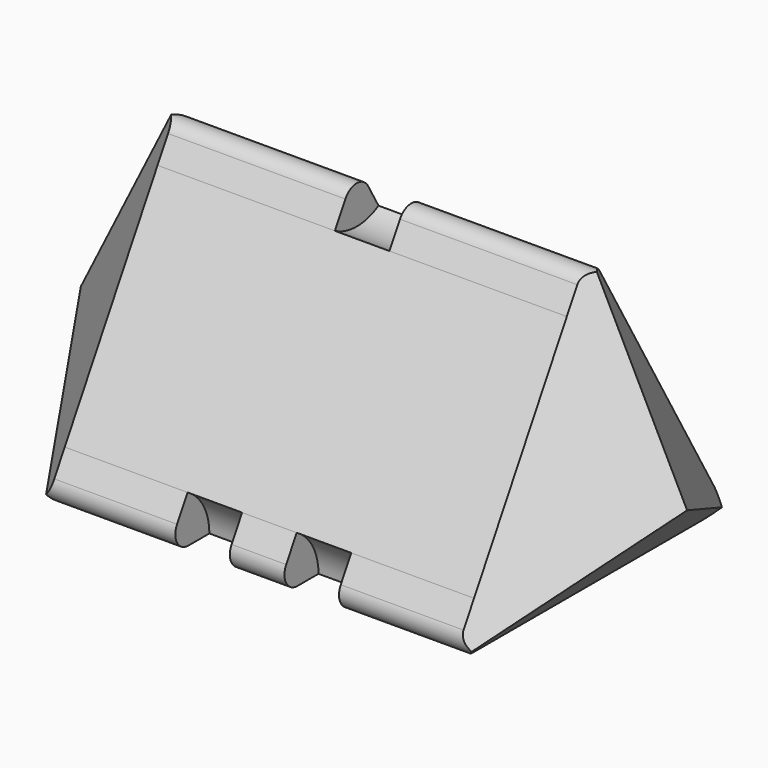
from build123d import *

# Parameters (mm, degrees)
F1_DEPTH    = 15
F4_T1_DEPTH = 20.1961524227
F5_START    = 6.5
F5_DEPTH    = 2
F6_START    = 4.5
F6_DEPTH    = 2
F7_START    = 8.5
F7_DEPTH    = 2
F8_START    = 2.5
F8_DEPTH    = 2
F9_START    = 6.5
F9_DEPTH    = 2
F10_START   = 10.5
F10_DEPTH   = 2


# Not quite as in the source:
# - a fillet or chamfer that OpenCascade refuses, or shapes differently, is made with other operations: its cross-section is extruded or revolved along the edge and cut away or added
# - an extrude whose draft closes it to a point is written as a loft to that point
# - a feature names something its author has since deleted; it is built from what else it names


with BuildPart() as f1:
    # F0 (on Right) → F1 (new body)
    with BuildSketch(Plane.YZ):
        with BuildLine():
            Line((4.25, 2.1650635095), (6.25, 2.1650635095))
            Line((6.25, 2.1650635095), (5.25, 3.897114317))
            ThreePointArc((5.25, 3.897114317), (4.5179491924, 3.1650635095), (4.25, 2.1650635095))
        make_face()
        with BuildLine():
            ThreePointArc((4.25, 2.1650635095), (4.5179491924, 3.1650635095), (5.25, 3.897114317))
            Line((5.25, 3.897114317), (1, 11.2583302492))
            ThreePointArc((1, 11.2583302492), (0, 10.9903810568), (-1, 11.2583302492))
            Line((-1, 11.2583302492), (-5.25, 3.897114317))
            ThreePointArc((-5.25, 3.897114317), (-4.5179491924, 3.1650635095), (-4.25, 2.1650635095))
            Line((-4.25, 2.1650635095), (4.25, 2.1650635095))
        make_face()
        with BuildLine():
            ThreePointArc((-1, 11.2583302492), (0, 10.9903810568), (1, 11.2583302492))
            Line((1, 11.2583302492), (0, 12.9903810568))
            Line((0, 12.9903810568), (-1, 11.2583302492))
        make_face()
        with BuildLine():
            Line((-6.25, 2.1650635095), (-4.25, 2.1650635095))
            ThreePointArc((-4.25, 2.1650635095), (-4.5179491924, 3.1650635095), (-5.25, 3.897114317))
            Line((-5.25, 3.897114317), (-6.25, 2.1650635095))
        make_face()
    extrude(amount=F1_DEPTH)

    # F1_face (on face) → F2 section 0
    with BuildSketch(Plane(origin=(0, 0, 5.7735026919), x_dir=(0, 1, 0), z_dir=(-1, 0, 0)), mode=Mode.PRIVATE) as f2_s0:
        Polygon((0, -7.2168783649), (6.25, 3.6084391824), (-6.25, 3.6084391824), align=None)
    loft([f2_s0.sketch, Vertex(-3.6084391824, 0, 5.7735026919)], ruled=True)

    # F1_face1 (on face) → F3 section 0
    with BuildSketch(Plane(origin=(15, 0, 5.7735026919), x_dir=(0, 1, 0), z_dir=(1, 0, 0)), mode=Mode.PRIVATE) as f3_s0:
        Polygon((6.25, -3.6084391824), (0, 7.2168783649), (-6.25, -3.6084391824), align=None)
    loft([f3_s0.sketch, Vertex(18.6084391824, 0, 5.7735026919)], ruled=True)

    # F4: fillet of radius 0.6 on 3 edges, made by hand

    # F4_s2 → F4_t1 (cut)
    with BuildSketch(Plane.YZ.offset(-2.5980762114)):
        with BuildLine():
            ThreePointArc((0.5196152423, 12.0903810568), (0, 12.3903810568), (-0.5196152423, 12.0903810568))
            Line((-0.5196152423, 12.0903810568), (0, 12.9903810568))
            Line((0, 12.9903810568), (0.5196152423, 12.0903810568))
        make_face()
        with BuildLine():
            ThreePointArc((-5.2107695155, 2.1650635095), (-5.7303847577, 2.4650635095), (-5.7303847577, 3.0650635095))
            Line((-5.7303847577, 3.0650635095), (-6.25, 2.1650635095))
            Line((-6.25, 2.1650635095), (-5.2107695155, 2.1650635095))
        make_face()
        with BuildLine():
            ThreePointArc((5.7303847577, 3.0650635095), (5.7303847577, 2.4650635095), (5.2107695155, 2.1650635095))
            Line((5.2107695155, 2.1650635095), (6.25, 2.1650635095))
            Line((6.25, 2.1650635095), (5.7303847577, 3.0650635095))
        make_face()
    extrude(amount=F4_T1_DEPTH, mode=Mode.SUBTRACT)

    # F0 (on Right) → F5 (cut)
    with BuildSketch(Plane.YZ.offset(F5_START)):
        with BuildLine():
            ThreePointArc((-1, 11.2583302492), (0, 10.9903810568), (1, 11.2583302492))
            Line((1, 11.2583302492), (0, 12.9903810568))
            Line((0, 12.9903810568), (-1, 11.2583302492))
        make_face()
    extrude(amount=F5_DEPTH, mode=Mode.SUBTRACT)

    # F0 (on Right) → F6 (cut)
    with BuildSketch(Plane.YZ.offset(F6_START)):
        with BuildLine():
            Line((-6.25, 2.1650635095), (-4.25, 2.1650635095))
            ThreePointArc((-4.25, 2.1650635095), (-4.5179491924, 3.1650635095), (-5.25, 3.897114317))
            Line((-5.25, 3.897114317), (-6.25, 2.1650635095))
        make_face()
    extrude(amount=F6_DEPTH, mode=Mode.SUBTRACT)

    # F0 (on Right) → F7 (cut)
    with BuildSketch(Plane.YZ.offset(F7_START)):
        with BuildLine():
            Line((-6.25, 2.1650635095), (-4.25, 2.1650635095))
            ThreePointArc((-4.25, 2.1650635095), (-4.5179491924, 3.1650635095), (-5.25, 3.897114317))
            Line((-5.25, 3.897114317), (-6.25, 2.1650635095))
        make_face()
    extrude(amount=F7_DEPTH, mode=Mode.SUBTRACT)

    # F0 (on Right) → F8 (cut)
    with BuildSketch(Plane.YZ.offset(F8_START)):
        with BuildLine():
            Line((4.25, 2.1650635095), (6.25, 2.1650635095))
            Line((6.25, 2.1650635095), (5.25, 3.897114317))
            ThreePointArc((5.25, 3.897114317), (4.5179491924, 3.1650635095), (4.25, 2.1650635095))
        make_face()
    extrude(amount=F8_DEPTH, mode=Mode.SUBTRACT)

    # F0 (on Right) → F9 (cut)
    with BuildSketch(Plane.YZ.offset(F9_START)):
        with BuildLine():
            Line((4.25, 2.1650635095), (6.25, 2.1650635095))
            Line((6.25, 2.1650635095), (5.25, 3.897114317))
            ThreePointArc((5.25, 3.897114317), (4.5179491924, 3.1650635095), (4.25, 2.1650635095))
        make_face()
    extrude(amount=F9_DEPTH, mode=Mode.SUBTRACT)

    # F0 (on Right) → F10 (cut)
    with BuildSketch(Plane.YZ.offset(F10_START)):
        with BuildLine():
            Line((4.25, 2.1650635095), (6.25, 2.1650635095))
            Line((6.25, 2.1650635095), (5.25, 3.897114317))
            ThreePointArc((5.25, 3.897114317), (4.5179491924, 3.1650635095), (4.25, 2.1650635095))
        make_face()
    extrude(amount=F10_DEPTH, mode=Mode.SUBTRACT)


solid = f1.part
